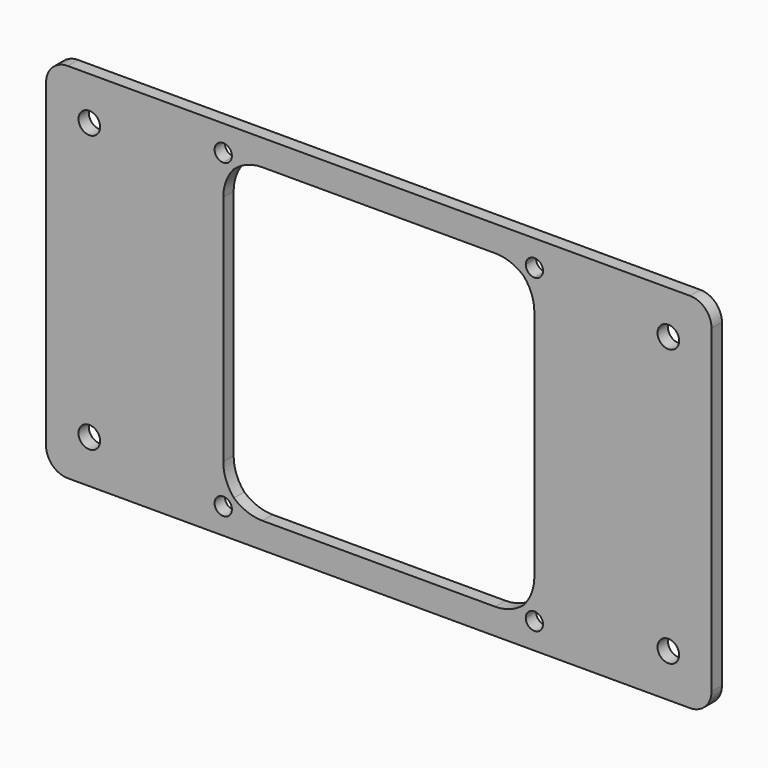
from build123d import *

# Parameters (mm, degrees)
F0_R        = 2.5
F1_DEPTH    = 3
F2_T1_DEPTH = 3


# Not quite as in the source:
# - a fillet or chamfer that OpenCascade refuses, or shapes differently, is made with other operations: its cross-section is extruded or revolved along the edge and cut away or added


with BuildPart() as f1:
    # F0 (on Front) → F1 (new body)
    with BuildSketch(Plane.XZ):
        with BuildLine():
            Line((-85.7558696013, 2.2170336112), (-85.7558696013, -11.7829663888))
            Line((-85.7558696013, -11.7829663888), (-85.7558696013, -26.7829663888))
            ThreePointArc((-85.7558696013, -26.7829663888), (-84.2914035073, -30.3185002947), (-80.7558696013, -31.7829663888))
            Line((-80.7558696013, -31.7829663888), (-70.7558696013, -31.7829663888))
            Line((-70.7558696013, -31.7829663888), (53.2441303987, -31.7829663888))
            Line((53.2441303987, -31.7829663888), (63.2441303987, -31.7829663888))
            ThreePointArc((63.2441303987, -31.7829663888), (66.7796643046, -30.3185002947), (68.2441303987, -26.7829663888))
            Line((68.2441303987, -26.7829663888), (68.2441303987, -17.7829663888))
            Line((68.2441303987, -17.7829663888), (68.2441303987, -11.7829663888))
            Line((68.2441303987, -11.7829663888), (68.2441303987, -2.7829663888))
            Line((68.2441303987, -2.7829663888), (68.2441303987, 2.2170336112))
            Line((68.2441303987, 2.2170336112), (68.2441303987, 32.2170336112))
            Line((68.2441303987, 32.2170336112), (68.2441303987, 47.2170336112))
            ThreePointArc((68.2441303987, 47.2170336112), (66.7796643046, 50.7525675171), (63.2441303987, 52.2170336112))
            Line((63.2441303987, 52.2170336112), (53.2441303987, 52.2170336112))
            Line((53.2441303987, 52.2170336112), (-70.7558696013, 52.2170336112))
            Line((-70.7558696013, 52.2170336112), (-80.7558696013, 52.2170336112))
            ThreePointArc((-80.7558696013, 52.2170336112), (-84.2914035073, 50.7525675171), (-85.7558696013, 47.2170336112))
            Line((-85.7558696013, 47.2170336112), (-85.7558696013, 32.2170336112))
            Line((-85.7558696013, 32.2170336112), (-85.7558696013, 2.2170336112))
        make_face()
        with Locations((-75.7558696013, -21.7829663888)):
            Circle(F0_R, mode=Mode.SUBTRACT)
        with BuildLine():
            ThreePointArc((-44.7558696013, 42.7170336112), (-47.2307433355, 48.6919073454), (-41.2558696013, 46.2170336112))
            Line((-41.2558696013, 46.2170336112), (23.7441303987, 46.2170336112))
            ThreePointArc((23.7441303987, 46.2170336112), (27.2441303987, 49.7170336112), (30.7441303987, 46.2170336112))
            ThreePointArc((30.7441303987, 46.2170336112), (29.7190041328, 43.7421598771), (27.2441303987, 42.7170336112))
            Line((27.2441303987, 42.7170336112), (27.2441303987, -22.2829663888))
            ThreePointArc((27.2441303987, -22.2829663888), (29.7190041328, -23.3080926546), (30.7441303987, -25.7829663888))
            ThreePointArc((30.7441303987, -25.7829663888), (27.2441303987, -29.2829663888), (23.7441303987, -25.7829663888))
            Line((23.7441303987, -25.7829663888), (-41.2558696013, -25.7829663888))
            ThreePointArc((-41.2558696013, -25.7829663888), (-47.2307433355, -28.2578401229), (-44.7558696013, -22.2829663888))
            Line((-44.7558696013, -22.2829663888), (-44.7558696013, 42.7170336112))
        make_face(mode=Mode.SUBTRACT)
        with Locations((58.2441303987, -21.7829663888)):
            Circle(F0_R, mode=Mode.SUBTRACT)
        with Locations((-75.7558696013, 42.2170336112)):
            Circle(F0_R, mode=Mode.SUBTRACT)
        with Locations((58.2441303987, 42.2170336112)):
            Circle(F0_R, mode=Mode.SUBTRACT)
        with BuildLine():
            ThreePointArc((-44.7558696013, 44.2170336112), (-46.1700831637, 47.6312471736), (-42.7558696013, 46.2170336112))
            Line((-42.7558696013, 46.2170336112), (-41.2558696013, 46.2170336112))
            ThreePointArc((-41.2558696013, 46.2170336112), (-47.2307433355, 48.6919073454), (-44.7558696013, 42.7170336112))
            Line((-44.7558696013, 42.7170336112), (-44.7558696013, 44.2170336112))
        make_face()
        with BuildLine():
            Line((-41.2558696013, 46.2170336112), (-42.7558696013, 46.2170336112))
            ThreePointArc((-42.7558696013, 46.2170336112), (-43.341656039, 44.8028200488), (-44.7558696013, 44.2170336112))
            Line((-44.7558696013, 44.2170336112), (-44.7558696013, 42.7170336112))
            ThreePointArc((-44.7558696013, 42.7170336112), (-42.2809958672, 43.7421598771), (-41.2558696013, 46.2170336112))
        make_face()
        with BuildLine():
            Line((-44.7558696013, -23.7829663888), (-44.7558696013, -22.2829663888))
            ThreePointArc((-44.7558696013, -22.2829663888), (-47.2307433355, -28.2578401229), (-41.2558696013, -25.7829663888))
            Line((-41.2558696013, -25.7829663888), (-42.7558696013, -25.7829663888))
            ThreePointArc((-42.7558696013, -25.7829663888), (-46.1700831637, -27.1971799512), (-44.7558696013, -23.7829663888))
        make_face()
        with BuildLine():
            ThreePointArc((-41.2558696013, -25.7829663888), (-42.2809958672, -23.3080926546), (-44.7558696013, -22.2829663888))
            Line((-44.7558696013, -22.2829663888), (-44.7558696013, -23.7829663888))
            ThreePointArc((-44.7558696013, -23.7829663888), (-43.341656039, -24.3687528264), (-42.7558696013, -25.7829663888))
            Line((-42.7558696013, -25.7829663888), (-41.2558696013, -25.7829663888))
        make_face()
        with BuildLine():
            Line((27.2441303987, -23.7829663888), (27.2441303987, -22.2829663888))
            ThreePointArc((27.2441303987, -22.2829663888), (24.7692566645, -23.3080926546), (23.7441303987, -25.7829663888))
            Line((23.7441303987, -25.7829663888), (25.2441303987, -25.7829663888))
            ThreePointArc((25.2441303987, -25.7829663888), (25.8299168363, -24.3687528264), (27.2441303987, -23.7829663888))
        make_face()
        with BuildLine():
            ThreePointArc((30.7441303987, -25.7829663888), (29.7190041328, -23.3080926546), (27.2441303987, -22.2829663888))
            Line((27.2441303987, -22.2829663888), (27.2441303987, -23.7829663888))
            ThreePointArc((27.2441303987, -23.7829663888), (28.658343961, -24.3687528264), (29.2441303987, -25.7829663888))
            ThreePointArc((29.2441303987, -25.7829663888), (27.2441303987, -27.7829663888), (25.2441303987, -25.7829663888))
            Line((25.2441303987, -25.7829663888), (23.7441303987, -25.7829663888))
            ThreePointArc((23.7441303987, -25.7829663888), (27.2441303987, -29.2829663888), (30.7441303987, -25.7829663888))
        make_face()
        with BuildLine():
            Line((25.2441303987, 46.2170336112), (23.7441303987, 46.2170336112))
            ThreePointArc((23.7441303987, 46.2170336112), (24.7692566645, 43.7421598771), (27.2441303987, 42.7170336112))
            Line((27.2441303987, 42.7170336112), (27.2441303987, 44.2170336112))
            ThreePointArc((27.2441303987, 44.2170336112), (25.8299168363, 44.8028200488), (25.2441303987, 46.2170336112))
        make_face()
        with BuildLine():
            ThreePointArc((30.7441303987, 46.2170336112), (27.2441303987, 49.7170336112), (23.7441303987, 46.2170336112))
            Line((23.7441303987, 46.2170336112), (25.2441303987, 46.2170336112))
            ThreePointArc((25.2441303987, 46.2170336112), (27.2441303987, 48.2170336112), (29.2441303987, 46.2170336112))
            ThreePointArc((29.2441303987, 46.2170336112), (28.658343961, 44.8028200488), (27.2441303987, 44.2170336112))
            Line((27.2441303987, 44.2170336112), (27.2441303987, 42.7170336112))
            ThreePointArc((27.2441303987, 42.7170336112), (29.7190041328, 43.7421598771), (30.7441303987, 46.2170336112))
        make_face()
    extrude(amount=F1_DEPTH)

    # F2: fillet of radius 10 on 8 edges, made by hand

    # F2_s2 → F2_t1 (join)
    with BuildSketch(Plane.XZ):
        with BuildLine():
            ThreePointArc((24.6515378061, 43.8657650921), (26.5734946341, 40.7482665367), (27.2441303987, 37.1478550376))
            Line((27.2441303987, 37.1478550376), (27.2441303987, 42.7170336112))
            ThreePointArc((27.2441303987, 42.7170336112), (25.8262869335, 43.0170773758), (24.6515378061, 43.8657650921))
        make_face()
        with BuildLine():
            ThreePointArc((18.1749518251, 46.2170336112), (21.7753633242, 45.5463978466), (24.8928618796, 43.6244410186))
            ThreePointArc((24.8928618796, 43.6244410186), (24.0441741633, 44.7991901461), (23.7441303987, 46.2170336112))
            Line((23.7441303987, 46.2170336112), (18.1749518251, 46.2170336112))
        make_face()
        with BuildLine():
            ThreePointArc((-42.4046010823, 43.6244410186), (-39.2871025268, 45.5463978466), (-35.6866910277, 46.2170336112))
            Line((-35.6866910277, 46.2170336112), (-41.2558696013, 46.2170336112))
            ThreePointArc((-41.2558696013, 46.2170336112), (-41.5559133659, 44.7991901461), (-42.4046010823, 43.6244410186))
        make_face()
        with BuildLine():
            ThreePointArc((-42.1632770087, 43.8657650921), (-44.0852338368, 40.7482665367), (-44.7558696013, 37.1478550376))
            Line((-44.7558696013, 37.1478550376), (-44.7558696013, 42.7170336112))
            ThreePointArc((-44.7558696013, 42.7170336112), (-43.3380261362, 43.0170773758), (-42.1632770087, 43.8657650921))
        make_face()
        with BuildLine():
            ThreePointArc((-42.1632770087, -23.4316978697), (-44.0852338368, -20.3141993143), (-44.7558696013, -16.7137878152))
            Line((-44.7558696013, -16.7137878152), (-44.7558696013, -22.2829663888))
            ThreePointArc((-44.7558696013, -22.2829663888), (-43.3380261362, -22.5830101534), (-42.1632770087, -23.4316978697))
        make_face()
        with BuildLine():
            ThreePointArc((-35.6866910277, -25.7829663888), (-39.2871025268, -25.1123306242), (-42.4046010823, -23.1903737962))
            ThreePointArc((-42.4046010823, -23.1903737962), (-41.5559133659, -24.3651229237), (-41.2558696013, -25.7829663888))
            Line((-41.2558696013, -25.7829663888), (-35.6866910277, -25.7829663888))
        make_face()
        with BuildLine():
            ThreePointArc((27.2441303987, -16.7137878152), (26.5734946341, -20.3141993143), (24.6515378061, -23.4316978697))
            ThreePointArc((24.6515378061, -23.4316978697), (25.8262869335, -22.5830101534), (27.2441303987, -22.2829663888))
            Line((27.2441303987, -22.2829663888), (27.2441303987, -16.7137878152))
        make_face()
        with BuildLine():
            ThreePointArc((24.8928618796, -23.1903737962), (21.7753633242, -25.1123306242), (18.1749518251, -25.7829663888))
            Line((18.1749518251, -25.7829663888), (23.7441303987, -25.7829663888))
            ThreePointArc((23.7441303987, -25.7829663888), (24.0441741633, -24.3651229237), (24.8928618796, -23.1903737962))
        make_face()
    extrude(amount=F2_T1_DEPTH)


solid = f1.part
